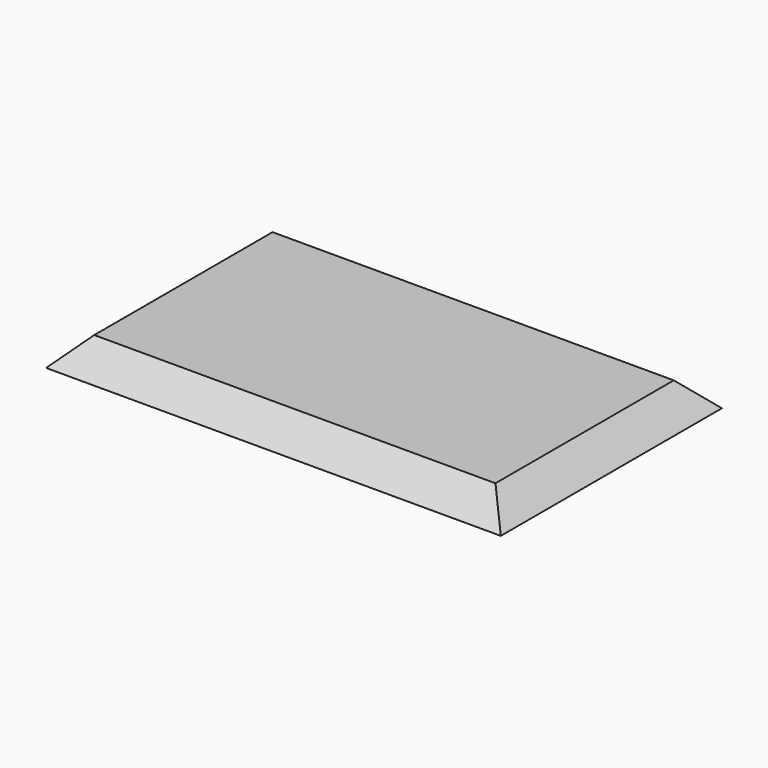
from build123d import *

# Parameters (mm, degrees)
F0_W     = 102
F0_H     = 62
F1_DEPTH = 6
F2_SIZE  = 5.99999


# Not quite as in the source:
# - a fillet or chamfer is up to 0.001 mm smaller than in the source, because OpenCascade refuses the exact size


with BuildPart() as f1:
    # F0 (on Top) → F1 (new body)
    with BuildSketch(Plane.XY):
        with Locations((51, 31)):
            Rectangle(F0_W, F0_H)
    extrude(amount=F1_DEPTH)

    # F2 (size 6 in the source; OpenCascade refuses exactly that, so slightly less here)
    f2_edges = [f1.edges().sort_by_distance(p)[0] for p in [
        (51, 0, 6),
        (102, 31, 6),
        (51, 62, 6),
        (0, 31, 6),
    ]]
    chamfer(f2_edges, length=F2_SIZE)


solid = f1.part
